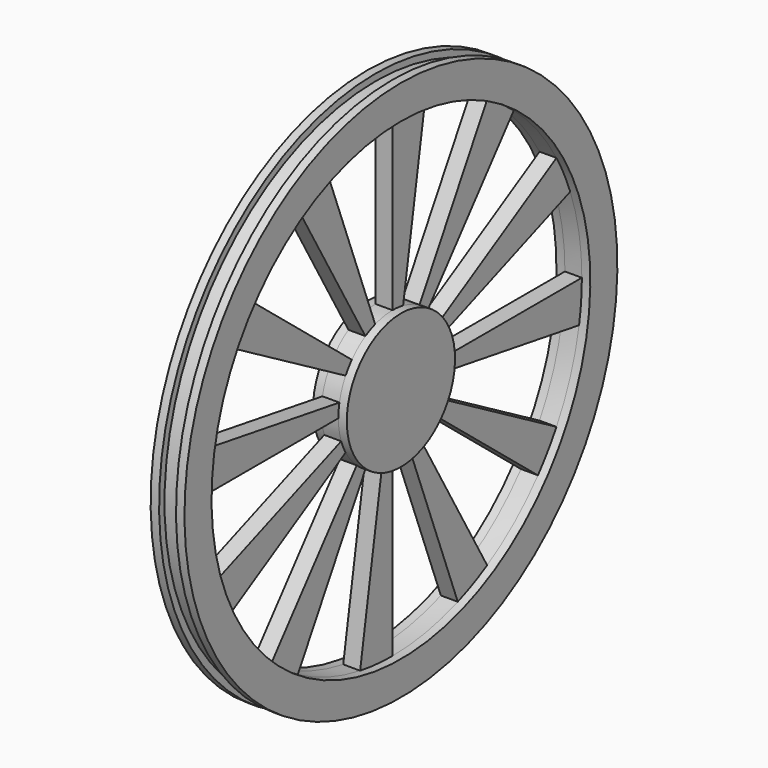
from build123d import *
from build123d import SkipClean  # not in build123d's __all__

# Parameters (mm, degrees)
F3_DEPTH        = 2.5
F3_COPIES_COUNT = 12


# Not quite as in the source:
# - after a boolean that leaves OpenCascade's solid faulty, fix() repairs it
# - a pattern or mirror of a feature is missing from the dataset's text; its kind, count and spacing are read off the source's solid


with BuildPart() as f1:
    # F0 (on Front) → F1 (revolve)
    with BuildSketch(Plane.XZ):
        Polygon((-5, -20), (0, -20), (0, -10), (-1.25, -10), (-1.25, 15), (0, 15), (0, 20), (-1.25, 20), (-1.25, 19), (-3.75, 19), (-3.75, 20), (-5, 20), (-5, 15), (-3.75, 15), (-3.75, -10), (-5, -10), align=None)
    revolve(axis=Axis((-2.5, 0, -20), (-1, 0, 0)))

    # F2 (on face) → F3 (cut, through all)
    with BuildSketch(Plane.YZ.offset(-1.25)):
        with BuildLine():
            Line((0, -10), (0, 15))
            ThreePointArc((0, 15), (-6.1307239653, 14.4588772838), (-12.0718779875, 12.8522413521))
            Line((-12.0718779875, 12.8522413521), (-3.1961564517, -10.5245272447))
            ThreePointArc((-3.1961564517, -10.5245272447), (-1.6194555331, -10.1320030515), (0, -10))
        make_face()
    with SkipClean():  # cleaning this boolean's faces spoils the solid; the shape is the same uncleaned
        f3 = extrude(amount=-F3_DEPTH, mode=Mode.SUBTRACT)

    # F3_copies: F3 ×12 about axis
    f3_copies_axis = Axis((0, 0, -20), (1, 0, 0))
    for i in range(1, F3_COPIES_COUNT):
        add(f3.rotate(f3_copies_axis, i * 360 / F3_COPIES_COUNT), clean=False, mode=Mode.SUBTRACT)

    add(f1.part.fix(), mode=Mode.REPLACE)


solid = f1.part
